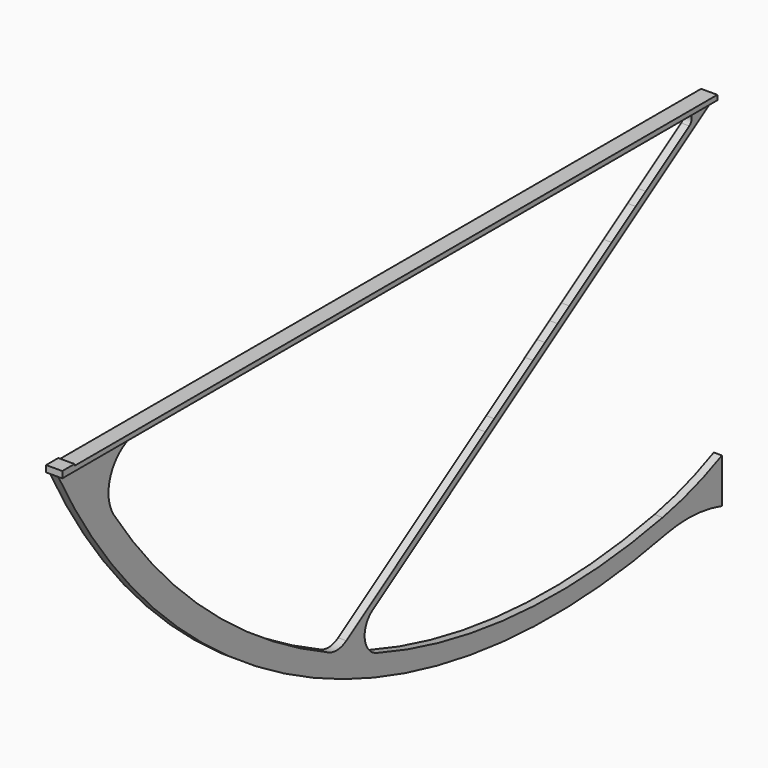
from build123d import *

# Parameters (mm, degrees)
F0_W        = 10
F0_H        = 3
F1_DEPTH    = 505
F3_DEPTH    = 2.5
F4_W        = 10
F4_H        = 9.3853771687
F5_DEPTH    = 1
F6_R        = 13.8620559507
F7_T1_DEPTH = 5
F8_T1_DEPTH = 5
F9_T1_DEPTH = 5
F10_R       = 3.9335934118


# Not quite as in the source:
# - a fillet or chamfer that OpenCascade refuses, or shapes differently, is made with other operations: its cross-section is extruded or revolved along the edge and cut away or added


with BuildPart() as f1:
    # F0 (on Front) → F1 (new body)
    with BuildSketch(Plane.XZ):
        with Locations((0, -9.24)):
            Rectangle(F0_W, F0_H)
    extrude(amount=F1_DEPTH)

    # F2 (on Right) → F3 (join, symmetric)
    with BuildSketch(Plane.YZ):
        with BuildLine():
            Line((-485, -10.74), (-505, -10.74))
            ThreePointArc((-505, -10.74), (-493.7857076195, -12.9341617837), (-482.5908295993, -15.2253199277))
            ThreePointArc((-482.5908295993, -15.2253199277), (-483.8023342329, -12.9863765535), (-485, -10.74))
        make_face()
        with BuildLine():
            ThreePointArc((-482.5908295993, -15.2253199277), (-493.7857076195, -12.9341617837), (-505, -10.74))
            ThreePointArc((-505, -10.74), (-295.8735946629, -205.4541731306), (-10.8822178841, -226.1272906733))
            Line((-10.8822178841, -226.1272906733), (-10.8822178841, -215.5293727716))
            ThreePointArc((-10.8822178841, -215.5293727716), (-149.5821295238, -229.2858372659), (-284.9469559253, -196.0703351995))
            ThreePointArc((-284.9469559253, -196.0703351995), (-287.1338212994, -195.111371401), (-289.3150994302, -194.1397657983))
            ThreePointArc((-289.3150994302, -194.1397657983), (-400.6140653387, -120.5204756417), (-482.5908295993, -15.2253199277))
        make_face()
        with BuildLine():
            Line((-175.5948523726, -120.1757838434), (-289.3150994302, -194.1397657983))
            ThreePointArc((-289.3150994302, -194.1397657983), (-287.1338212994, -195.111371401), (-284.9469559253, -196.0703351995))
            Line((-284.9469559253, -196.0703351995), (-164.6339868931, -117.8184275517))
            Line((-164.6339868931, -117.8184275517), (0, -10.74))
            Line((0, -10.74), (-7.3364102674, -10.74))
            Line((-7.3364102674, -10.74), (-52.0490416838, -39.8212265081))
            Line((-52.0490416838, -39.8212265081), (-59.8008067738, -44.8629972399))
            Line((-59.8008067738, -44.8629972399), (-69.1519232492, -50.9449907999))
            Line((-69.1519232492, -50.9449907999), (-78.2792164974, -56.881409077))
            Line((-78.2792164974, -56.881409077), (-110.8941655597, -78.0942675285))
            Line((-110.8941655597, -78.0942675285), (-120.0217871415, -84.0308993547))
            Line((-120.0217871415, -84.0308993547), (-129.6997254261, -90.3254587772))
            Line((-129.6997254261, -90.3254587772), (-138.8888255597, -96.3020764336))
            Line((-138.8888255597, -96.3020764336), (-168.8523264487, -115.7904252229))
            Line((-168.8523264487, -115.7904252229), (-175.5948523726, -120.1757838434))
        make_face()
        Polygon((-10.8822178841, -215.5293727716), (-10.8822178841, -226.1272906733), (6.6898409277, -234.5661967993), (6.6898409277, -207.0904666456), align=None)
    extrude(amount=F3_DEPTH, both=True)

    # F4 (on face) → F5 (join)
    with BuildSketch(Plane.XY.offset(-7.74)):
        with Locations((0, -500.3073114157)):
            Rectangle(F4_W, F4_H)
    extrude(amount=F5_DEPTH)

    # F6
    f6_edges = [f1.edges().sort_by_distance(p)[0] for p in [
        (0, -284.946956, -196.070335),
        (0, -289.315099, -194.139766),
    ]]
    fillet(f6_edges, radius=F6_R)

    # F7: fillet of radius 24.5086487231 on 1 edges, made by hand

    # F7_s2 → F7_t1 (join)
    with BuildSketch(Plane.YZ.offset(-2.5)):
        with BuildLine():
            ThreePointArc((-441.73429524, -10.74), (-463.3828258275, -23.7588712825), (-462.0321746683, -48.9843668676))
            ThreePointArc((-462.0321746683, -48.9843668676), (-474.0334147231, -30.1728667078), (-485, -10.74))
            Line((-485, -10.74), (-441.73429524, -10.74))
        make_face()
    extrude(amount=F7_T1_DEPTH)

    # F8: fillet of radius 198.8084962623 on 1 edges, made by hand

    # F8_s2 → F8_t1 (join)
    with BuildSketch(Plane.YZ.offset(-2.5)):
        with BuildLine():
            ThreePointArc((-38.9541818345, -222.2094923529), (-15.6734102854, -216.0349668625), (6.6898409277, -207.0904666456))
            Line((6.6898409277, -207.0904666456), (-10.8822178841, -215.5293727716))
            ThreePointArc((-10.8822178841, -215.5293727716), (-24.8597763304, -219.11494661), (-38.9541818345, -222.2094923529))
        make_face()
    extrude(amount=F8_T1_DEPTH)

    # F9: fillet of radius 87.6851690928 on 1 edges, made by hand

    # F9_s2 → F9_t1 (join)
    with BuildSketch(Plane.YZ.offset(-2.5)):
        with BuildLine():
            ThreePointArc((6.6898409277, -234.5661967993), (-15.0768754349, -230.7023497098), (-37.1181822791, -232.4053024821))
            ThreePointArc((-37.1181822791, -232.4053024821), (-23.9509608314, -229.4720686048), (-10.8822178841, -226.1272906733))
            Line((-10.8822178841, -226.1272906733), (6.6898409277, -234.5661967993))
        make_face()
    extrude(amount=F9_T1_DEPTH)

    # F10
    f10_edges = [f1.edges().sort_by_distance(p)[0] for p in [
        (0, -7.33641, -10.74),
    ]]
    fillet(f10_edges, radius=F10_R)


solid = f1.part
